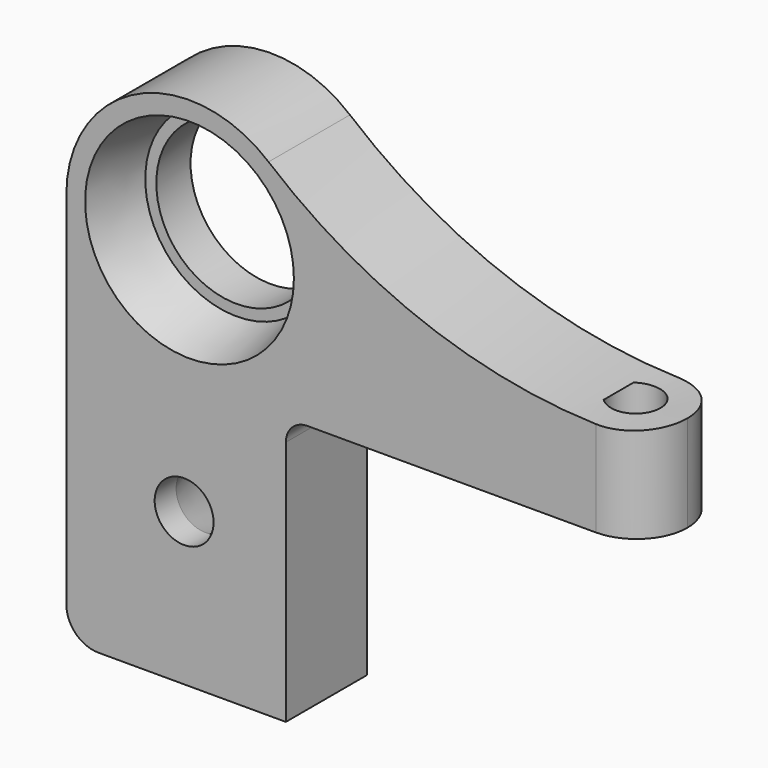
from build123d import *

# Parameters (mm, degrees)
F1_DEPTH       = 9.5
F2_R           = 7.5
F3_DEPTH       = 9.5
F4_R           = 8.5
F5_DEPTH       = 5.5
F6_R           = 9.75
F7_DEPTH       = 5.5
F7_TAPER       = 12.5
F7_DEPTH_BACK  = 25
F8_R           = 4.75
F9_R           = 4.74999
F10_R          = 3
F11_R          = 2
F13_R          = 2.35
F14_DEPTH      = 10
F16_R          = 2.75
F17_DEPTH      = 9.5
F18_R          = 5
F19_DEPTH      = 7
F19_TAPER      = 17.5
F19_DEPTH_BACK = 7


# Not quite as in the source:
# - a fillet or chamfer is up to 0.001 mm smaller than in the source, because OpenCascade refuses the exact size


with BuildPart() as f1:
    # F0 (on Front) → F1 (new body)
    with BuildSketch(Plane.XZ):
        with BuildLine():
            Line((0, 36.7), (0, 0))
            Line((0, 0), (20.5, 0))
            Line((20.5, 0), (20.5, 24.9898828528))
            Line((20.5, 24.9898828528), (54.2, 24.9898828528))
            Line((54.2, 24.9898828528), (54.2, 33.9898828528))
            ThreePointArc((54.2, 33.9898828528), (35.4283305629, 36.3418613979), (18.8835293674, 45.5166600298))
            ThreePointArc((18.8835293674, 45.5166600298), (6.6348477786, 47.1201868439), (0, 36.7))
        make_face()
    extrude(amount=-F1_DEPTH)

    # F2 (on Front) → F3 (cut)
    with BuildSketch(Plane.XZ):
        with Locations((11.5, 36.7)):
            Circle(F2_R)
    extrude(amount=-F3_DEPTH, mode=Mode.SUBTRACT)

    # F4 (on Front) → F5 (cut)
    with BuildSketch(Plane.XZ):
        with Locations((11.5, 36.7)):
            Circle(F4_R)
    extrude(amount=-F5_DEPTH, mode=Mode.SUBTRACT)

    # F6 (on Front) → F7 (cut, two sides)
    with BuildSketch(Plane.XZ) as f7_sk:
        with Locations((11.5, 36.7)):
            Circle(F6_R)
    extrude(amount=-F7_DEPTH, taper=F7_TAPER, mode=Mode.SUBTRACT)
    extrude(f7_sk.sketch, amount=F7_DEPTH_BACK, mode=Mode.SUBTRACT)

    # F8
    f8_edges = [f1.edges().sort_by_distance(p)[0] for p in [
        (54.2, 0, 29.489883),
    ]]
    fillet(f8_edges, radius=F8_R)

    # F9 (radius 4.75 in the source; OpenCascade refuses exactly that, so slightly less here)
    f9_edges = [f1.edges().sort_by_distance(p)[0] for p in [
        (54.2, 9.5, 29.489883),
    ]]
    fillet(f9_edges, radius=F9_R)

    # F10
    f10_edges = [f1.edges().sort_by_distance(p)[0] for p in [
        (0, 4.75, 0),
    ]]
    fillet(f10_edges, radius=F10_R)

    # F11
    f11_edges = [f1.edges().sort_by_distance(p)[0] for p in [
        (20.5, 4.75, 24.989883),
    ]]
    fillet(f11_edges, radius=F11_R)

    # F13 (on face) → F14 (cut)
    with BuildSketch(Plane.XY.offset(33.9898828528)):
        with Locations((49.1753853858, 4.9540796317)):
            Circle(F13_R)
    extrude(amount=-F14_DEPTH, mode=Mode.SUBTRACT)

    # F16 (on offset) → F17 (cut)
    with BuildSketch(Plane.XZ.offset(-9.5)):
        with Locations((11, 14.2)):
            Circle(F16_R)
    extrude(amount=F17_DEPTH, mode=Mode.SUBTRACT)

    # F18 (on offset) → F19 (cut, two sides)
    with BuildSketch(Plane.XZ.offset(-9.5)) as f19_sk:
        with Locations((11, 14.2)):
            Circle(F18_R)
    extrude(amount=F19_DEPTH, taper=F19_TAPER, mode=Mode.SUBTRACT)
    extrude(f19_sk.sketch, amount=-F19_DEPTH_BACK, mode=Mode.SUBTRACT)


solid = f1.part
